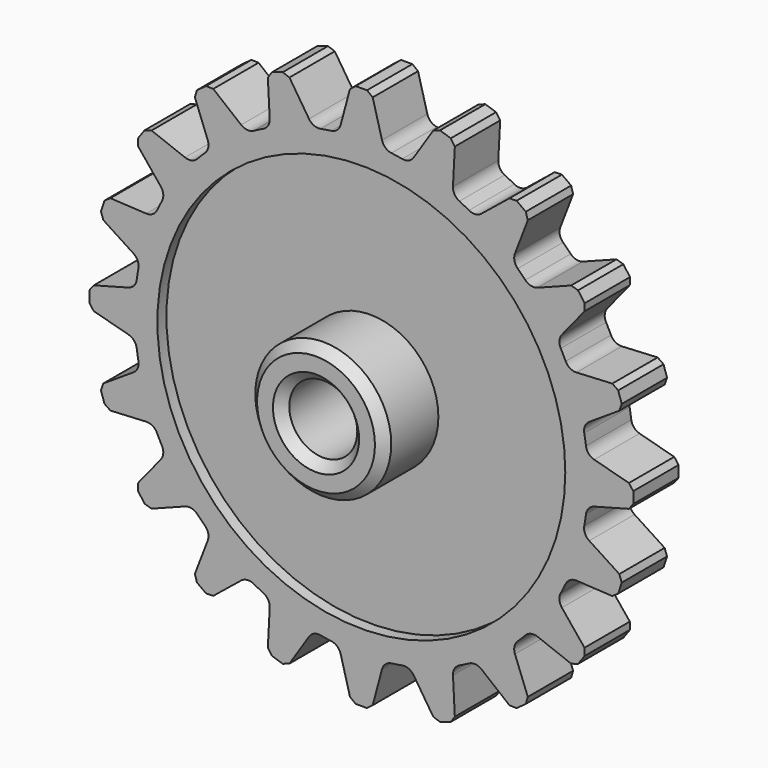
from build123d import *

# Parameters (mm, degrees)
F0_R            = 100
F1_DEPTH        = 25
F3_DEPTH        = 25
F3_COPIES_COUNT = 20
F4_SIZE         = 2
F5_R            = 5
F6_R            = 90
F7_DEPTH        = 5
F8_R            = 30
F9_DEPTH        = 30
F10_R           = 15
F11_DEPTH       = 50.001
F12_SIZE        = 4


# Not quite as in the source:
# - a pattern or mirror of a feature is missing from the dataset's text; its kind, count and spacing are read off the source's solid


with BuildPart() as f1:
    # F0 (on Front) → F1 (new body)
    with BuildSketch(Plane.XZ):
        Circle(F0_R)
    extrude(amount=F1_DEPTH)

    # F2 (on Front) → F3 (join)
    with BuildSketch(Plane.XZ):
        Polygon((4.5, 120), (-4.5, 120), (-9.9931095726, 99.4994359837), (9.9931095726, 99.4994359837), align=None)
    f3 = extrude(amount=F3_DEPTH)

    # F3_copies: F3 ×20 about axis
    f3_copies_axis = Axis((0, 0, 0), (0, 1, 0))
    for i in range(1, F3_COPIES_COUNT):
        add(f3.rotate(f3_copies_axis, i * 360 / F3_COPIES_COUNT))

    # F4
    f4_edges = [f1.edges().sort_by_distance(p)[0] for p in [
        (4.5, -12.5, 120),
        (-4.5, -12.5, 120),
        (-32.802285, -12.5, 115.517358),
        (115.517358, -12.5, 32.802285),
        (120, -12.5, 4.5),
        (120, -12.5, -4.5),
        (115.517358, -12.5, -32.802285),
        (112.736205, -12.5, -41.361794),
        (99.727073, -12.5, -66.893654),
        (94.437006, -12.5, -74.174807),
        (74.174807, -12.5, -94.437006),
        (66.893654, -12.5, -99.727073),
        (41.361794, -12.5, -112.736205),
        (32.802285, -12.5, -115.517358),
        (4.5, -12.5, -120),
        (-4.5, -12.5, -120),
        (-32.802285, -12.5, -115.517358),
        (-41.361794, -12.5, -112.736205),
        (-66.893654, -12.5, -99.727073),
        (-74.174807, -12.5, -94.437006),
        (-94.437006, -12.5, -74.174807),
        (-99.727073, -12.5, -66.893654),
        (-112.736205, -12.5, -41.361794),
        (-115.517358, -12.5, -32.802285),
        (-120, -12.5, -4.5),
        (-120, -12.5, 4.5),
        (-115.517358, -12.5, 32.802285),
        (-112.736205, -12.5, 41.361794),
        (-99.727073, -12.5, 66.893654),
        (-94.437006, -12.5, 74.174807),
        (-74.174807, -12.5, 94.437006),
        (-66.893654, -12.5, 99.727073),
        (32.802285, -12.5, 115.517358),
        (41.361794, -12.5, 112.736205),
        (66.893654, -12.5, 99.727073),
        (74.174807, -12.5, 94.437006),
        (94.437006, -12.5, 74.174807),
        (99.727073, -12.5, 66.893654),
        (112.736205, -12.5, 41.361794),
        (-41.361794, -12.5, 112.736205),
    ]]
    chamfer(f4_edges, length=F4_SIZE)

    # F5
    f5_edges = [f1.edges().sort_by_distance(p)[0] for p in [
        (9.99311, -12.5, 99.499436),
        (-9.99311, -12.5, 99.499436),
        (97.717628, -12.5, 21.243005),
        (99.499436, -12.5, 9.99311),
        (91.541546, -12.5, 40.251029),
        (86.370537, -12.5, 50.399706),
        (99.499436, -12.5, -9.99311),
        (97.717628, -12.5, -21.243005),
        (74.622932, -12.5, 66.568897),
        (66.568897, -12.5, 74.622932),
        (91.541546, -12.5, -40.251029),
        (86.370537, -12.5, -50.399706),
        (50.399706, -12.5, 86.370537),
        (40.251029, -12.5, 91.541546),
        (74.622932, -12.5, -66.568897),
        (66.568897, -12.5, -74.622932),
        (21.243005, -12.5, 97.717628),
        (50.399706, -12.5, -86.370537),
        (40.251029, -12.5, -91.541546),
        (-21.243005, -12.5, 97.717628),
        (21.243005, -12.5, -97.717628),
        (9.99311, -12.5, -99.499436),
        (-40.251029, -12.5, 91.541546),
        (-50.399706, -12.5, 86.370537),
        (-9.99311, -12.5, -99.499436),
        (-21.243005, -12.5, -97.717628),
        (-66.568897, -12.5, 74.622932),
        (-74.622932, -12.5, 66.568897),
        (-40.251029, -12.5, -91.541546),
        (-50.399706, -12.5, -86.370537),
        (-86.370537, -12.5, 50.399706),
        (-91.541546, -12.5, 40.251029),
        (-66.568897, -12.5, -74.622932),
        (-74.622932, -12.5, -66.568897),
        (-97.717628, -12.5, 21.243005),
        (-99.499436, -12.5, 9.99311),
        (-86.370537, -12.5, -50.399706),
        (-91.541546, -12.5, -40.251029),
        (-99.499436, -12.5, -9.99311),
        (-97.717628, -12.5, -21.243005),
    ]]
    fillet(f5_edges, radius=F5_R)

    # F6 (on face) → F7 (cut)
    with BuildSketch(Plane.XZ.offset(25)):
        Circle(F6_R)
    extrude(amount=-F7_DEPTH, mode=Mode.SUBTRACT)

    # F8 (on face) → F9 (join)
    with BuildSketch(Plane.XZ.offset(20)):
        Circle(F8_R)
    extrude(amount=F9_DEPTH)

    # F10 (on face) → F11 (cut, through all)
    with BuildSketch(Plane.XZ.offset(50)):
        Circle(F10_R)
    extrude(amount=-F11_DEPTH, mode=Mode.SUBTRACT)

    # F12
    f12_edges = [f1.edges().sort_by_distance(p)[0] for p in [
        (-30, -50, 0),
        (-15, -50, 0),
    ]]
    chamfer(f12_edges, length=F12_SIZE)


solid = f1.part
